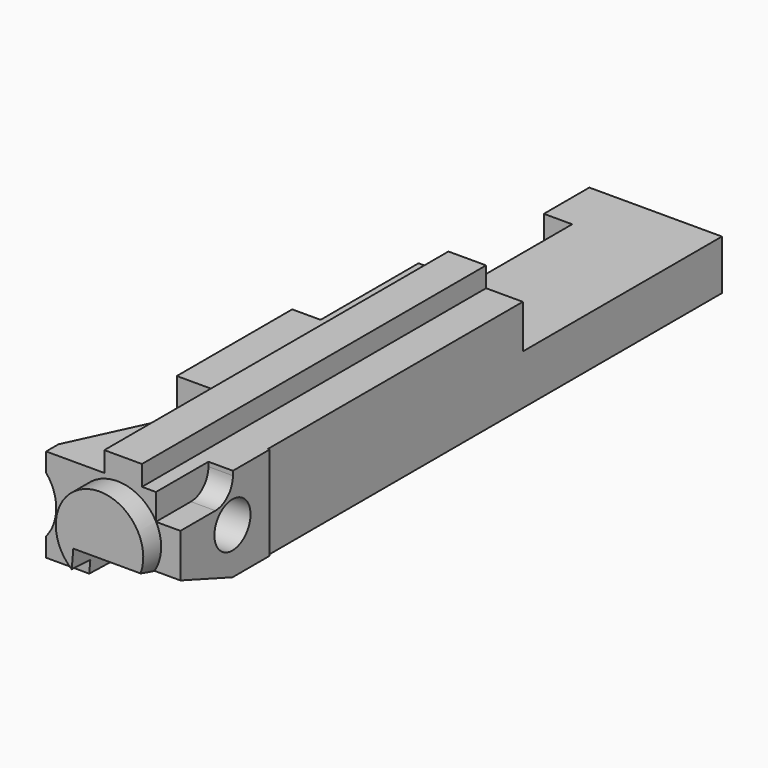
from build123d import *

# Parameters (mm, degrees)
F11_W           = 19.2532
F11_H           = 16.51
F12_DEPTH       = 98.6028
F0_W            = 8.4582
F0_H            = 2.921
F0_W_2          = 5.334
F13_DEPTH       = 98.6038
F14_W           = 36.1442
F14_H           = 6.35
F14_H_2         = 2.921
F2_DEPTH        = 19.2542
F15_W           = 5.4102
F15_H           = 9.8806
F15_W_2         = 4.1148
F15_H_2         = 45.6692
F3_DEPTH        = 16.511
F5_DEPTH        = 5.401076254
F4_R            = 6.35
F6_DEPTH        = 3.2512
F17_DEPTH       = 14.224
F7_T4_DEPTH     = 104.0831879802
F7_T10_DEPTH    = 104.0831879802
F7_S12_R        = 6.35
F7_T13_DEPTH    = 60
F18_DEPTH       = 0.254
F8_W            = 3.556
F8_H            = 9.525
F9_DEPTH        = 3.81
F19_R           = 3.175
F20_D           = 5.7658
F20_DEPTH       = 13.208
F20_CBORE_D     = 6.5532
F20_CBORE_DEPTH = 8.255
F20_TIP         = 1.7322210786


# Not quite as in the source:
# - a fillet or chamfer that OpenCascade refuses, or shapes differently, is made with other operations: its cross-section is extruded or revolved along the edge and cut away or added


with BuildPart() as f12:
    # F11 (on Front) → F12 (new body)
    with BuildSketch(Plane.XZ):
        with Locations((9.6266, -8.255)):
            Rectangle(F11_W, F11_H)
    extrude(amount=F12_DEPTH)

    # F0 (on face) → F13 (cut, through all)
    with BuildSketch(Plane.XZ.offset(98.6028)):
        with Locations((4.2291, -1.4605)):
            Rectangle(F0_W, F0_H)
        with Locations((16.5862, -1.4605)):
            Rectangle(F0_W_2, F0_H)
    extrude(amount=-F13_DEPTH, mode=Mode.SUBTRACT)

    # F14 (on face) → F2 (cut, through all)
    with BuildSketch(Plane(origin=(0, 0, 0), x_dir=(0, -1, 0), z_dir=(-1, 0, 0))):
        with Locations((18.0721, -6.096)):
            Rectangle(F14_W, F14_H)
        with Locations((18.0721, -1.4605)):
            Rectangle(F14_W, F14_H_2)
    extrude(amount=-F2_DEPTH, mode=Mode.SUBTRACT)

    # F15 (on face) → F3 (cut, through all)
    with BuildSketch(Plane(origin=(0, 0, -16.51), x_dir=(1, 0, 0), z_dir=(0, 0, -1))):
        Polygon((0, 96.3620113413), (0, 84.7598), (5.4102, 84.7598), align=None)
        with Locations((2.7051, 79.8195)):
            Rectangle(F15_W, F15_H)
        with Locations((2.0574, 31.0896)):
            Rectangle(F15_W_2, F15_H_2)
    extrude(amount=-F3_DEPTH, mode=Mode.SUBTRACT)

    # F4 (on face) → F5 (cut, through all)
    with BuildSketch(Plane.XZ.offset(98.6028)):
        with BuildLine():
            ThreePointArc((0, -13.7665703571), (1.093550911, -11.8624459294), (1.4732, -9.6997138609))
            ThreePointArc((1.4732, -9.6997138609), (1.093550911, -7.5369817925), (0, -5.6328573648))
            Line((0, -5.6328573648), (0, -13.7665703571))
        make_face()
    extrude(amount=-F5_DEPTH, mode=Mode.SUBTRACT)

    # F4 (on face) → F6 (join)
    with BuildSketch(Plane.XZ.offset(98.6028)):
        with Locations((10.3632, -9.6997138609)):
            Circle(F4_R)
    extrude(amount=F6_DEPTH)

    # F16 (on face) → F17 (cut)
    with BuildSketch(Plane.YZ.offset(19.2532)):
        Polygon((-89.154, -16.51), (-98.6028, -13.0709180505), (-98.6028, -16.51), align=None)
        Polygon((-98.6028, -13.0709180505), (-101.854, -11.8875780248), (-101.854, -16.51), (-98.6028, -16.51), align=None)
    extrude(amount=-F17_DEPTH, mode=Mode.SUBTRACT)

    # F7: chamfer of 1.524 x 17.4193997094 on 1 edges, made by hand


with BuildPart() as f7_tool2:
    # F7_s3 → F7_t4 (new body)
    with BuildSketch(Plane(origin=(0, -30.8656495765, 11.2341777071), x_dir=(1, 0, 0), z_dir=(0, -0.9396926208, 0.3420201433))):
        Polygon((5.0292, -63.4261887366), (6.5532, -46.0067890272), (5.0292, -46.0067890272), align=None)
    extrude(amount=F7_T4_DEPTH)

    split(bisect_by=Plane.XY.offset(-16.51), keep=Keep.TOP)

    split(bisect_by=Plane.XZ.offset(98.6028), keep=Keep.BOTTOM)


with BuildPart() as f12_1:
    add(f12.part)

    # F7_t1: union F7_tool2
    add(f7_tool2.part)


with BuildPart() as f7_tool8:
    # F7_s9 → F7_t10 (new body)
    with BuildSketch(Plane(origin=(0, -30.8656495765, 11.2341777071), x_dir=(1, 0, 0), z_dir=(0, -0.9396926208, 0.3420201433))):
        Polygon((5.0292, -63.4261887366), (6.5532, -46.0067890272), (5.0292, -46.0067890272), align=None)
    extrude(amount=F7_T10_DEPTH)

    split(bisect_by=Plane.XZ.offset(101.854), keep=Keep.BOTTOM)

    # F7_s12 → F7_t13 (intersect, symmetric)
    with BuildSketch(Plane.XZ.offset(98.5)):
        with Locations((10.3632, -9.6997138609)):
            Circle(F7_S12_R)
    extrude(amount=F7_T13_DEPTH, both=True, mode=Mode.INTERSECT)


with BuildPart() as f12_2:
    add(f12_1.part)

    # F7_t7: union F7_tool8
    add(f7_tool8.part)

    # F16 (on face) → F18 (join)
    with BuildSketch(Plane.YZ.offset(19.2532)):
        Polygon((-98.6028, -2.921), (-98.6028, -13.0709180505), (-89.154, -16.51), (-82.4484, -16.51), (-82.4484, -2.921), align=None)
    extrude(amount=F18_DEPTH)

    # F8 (on face) → F9 (cut)
    with BuildSketch(Plane.XY.offset(-2.921)):
        with Locations((17.7292, -93.8403)):
            Rectangle(F8_W, F8_H)
    extrude(amount=-F9_DEPTH, mode=Mode.SUBTRACT)

    # F19
    f19_edges = [f12_2.edges().sort_by_distance(p)[0] for p in [
        (17.7292, -89.0778, -6.731),
    ]]
    fillet(f19_edges, radius=F19_R)

    # F20
    with Locations(Plane.YZ.offset(19.5072)):
        with Locations((-89.154, -9.8044)):
            CounterBoreHole(F20_D / 2, F20_CBORE_D / 2, F20_CBORE_DEPTH, depth=F20_DEPTH)
            with Locations((0, 0, -(F20_DEPTH + F20_TIP / 2))):  # 118° drill point
                Cone(0, F20_D / 2, F20_TIP, mode=Mode.SUBTRACT)


solid = f12_2.part
